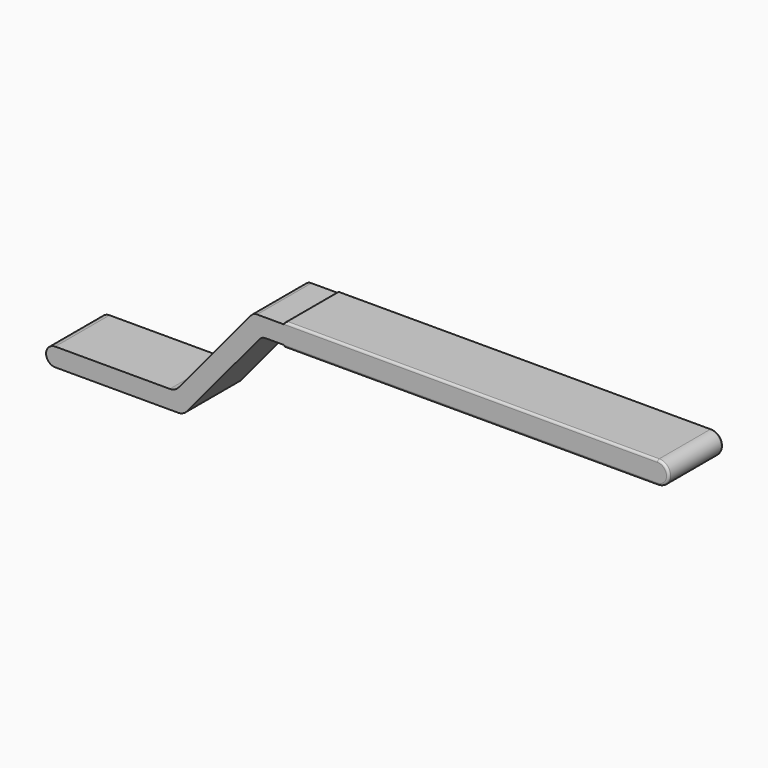
from build123d import *

# Parameters (mm, degrees)
F1_DEPTH = 30
F2_R     = 0.99999


# Not quite as in the source:
# - a fillet or chamfer is up to 0.001 mm smaller than in the source, because OpenCascade refuses the exact size


with BuildPart() as f1:
    # F0 (on Front) → F1 (new body)
    with BuildSketch(Plane.XZ):
        with BuildLine():
            Line((-63.6692684564, 20.8099257126), (-114.3268977837, 20.8099257126))
            ThreePointArc((-114.3268977837, 20.8099257126), (-118.3668602392, 16.7699632572), (-114.3268977837, 12.7300008017))
            Line((-114.3268977837, 12.7300008017), (-59.988057444, 12.7300008017))
            ThreePointArc((-59.988057444, 12.7300008017), (-57.8669121635, 13.2022262159), (-56.1464303666, 14.5297037219))
            Line((-56.1464303666, 14.5297037219), (-24.0653757294, 53.0397061037))
            ThreePointArc((-24.0653757294, 53.0397061037), (-22.8610384715, 53.9689403579), (-21.3762367753, 54.2994981479))
            Line((-21.3762367753, 54.2994981479), (-13.1770761366, 54.2994981479))
            Line((-13.1770761366, 54.2994981479), (-13.1770761366, 62.2994981479))
            Line((-13.1770761366, 62.2994981479), (-25.1240298515, 62.2994981479))
            ThreePointArc((-25.1240298515, 62.2994981479), (-26.6088315478, 61.9689403579), (-27.8131688056, 61.0397061037))
            Line((-27.8131688056, 61.0397061037), (-59.8276413791, 22.6096286329))
            ThreePointArc((-59.8276413791, 22.6096286329), (-61.548123176, 21.2821511269), (-63.6692684564, 20.8099257126))
        make_face()
        with BuildLine():
            Line((-13.1770761366, 63.2994981479), (-13.1770761366, 62.2994981479))
            Line((-13.1770761366, 62.2994981479), (-13.1770761366, 54.2994981479))
            Line((-13.1770761366, 54.2994981479), (-13.1770761366, 53.2994981479))
            Line((-13.1770761366, 53.2994981479), (151.8229238634, 53.2994981479))
            ThreePointArc((151.8229238634, 53.2994981479), (156.8229238634, 58.2994981479), (151.8229238634, 63.2994981479))
            Line((151.8229238634, 63.2994981479), (-13.1770761366, 63.2994981479))
        make_face()
    extrude(amount=F1_DEPTH)

    # F2 (radius 1 in the source; OpenCascade refuses exactly that, so slightly less here)
    f2_edges = [f1.edges().sort_by_distance(p)[0] for p in [
        (69.322924, 0, 63.299498),
        (69.322924, -30, 53.299498),
        (151.822924, -15, 63.299498),
        (151.822924, -15, 53.299498),
        (-13.177076, -15, 53.299498),
        (-13.177076, -15, 63.299498),
    ]]
    fillet(f2_edges, radius=F2_R)


solid = f1.part
